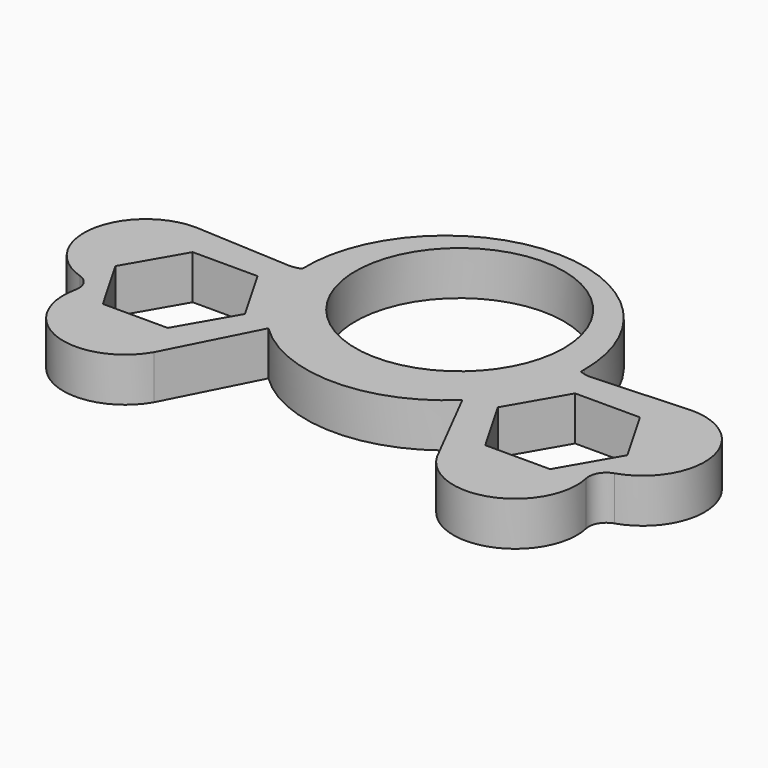
from build123d import *

# Parameters (mm, degrees)
F0_R     = 11.8128779822
F1_DEPTH = 5


with BuildPart() as f1:
    # F0 (on Top) → F1 (new body)
    with BuildSketch(Plane.XY):
        with BuildLine():
            ThreePointArc((-10.9877368692, -13.3584800376), (-14.4276328661, -8.4296575195), (-15.7757547816, -2.5722909453))
            ThreePointArc((-15.7757547816, -2.5722909453), (-16.4566838692, -2.7870228586), (-17.1690704864, -2.8347672253))
            Line((-17.1690704864, -2.8347672253), (-28.1587377075, -2.2588231712))
            ThreePointArc((-28.1587377075, -2.2588231712), (-35.0758085793, -8.184518487), (-30.2818924612, -15.9290715842))
            ThreePointArc((-30.2818924612, -15.9290715842), (-29.1564572976, -16.8348568451), (-28.9347418331, -18.2624049175))
            ThreePointArc((-28.9347418331, -18.2624049175), (-24.6247201691, -26.286334608), (-16.0343820545, -23.2588231712))
            Line((-16.0343820545, -23.2588231712), (-11.038330626, -13.4535201515))
            ThreePointArc((-11.038330626, -13.4535201515), (-11.0134601469, -13.4057731047), (-10.9877368692, -13.3584800376))
        make_face()
        Polygon((-29.0074426032, -12.5088231712), (-25.3354948912, -6.1488231712), (-17.9915994671, -6.1488231712), (-14.319651755, -12.5088231712), (-17.9915994671, -18.8688231712), (-25.3354948912, -18.8688231712), align=None, mode=Mode.SUBTRACT)
        with BuildLine():
            ThreePointArc((15.7758429715, -2.5697420135), (15.7828894553, -2.2975080655), (15.7852385163, -2.0251930691))
            ThreePointArc((15.7852385163, -2.0251930691), (13.4879848824, 6.1752958693), (7.264870736, 11.9889215374))
            ThreePointArc((7.264870736, 11.9889215374), (-8.4330311307, 11.3186347537), (-15.7757547816, -2.5722909453))
            ThreePointArc((-15.7757547816, -2.5722909453), (-14.4276328661, -8.4296575195), (-10.9877368692, -13.3584800376))
            ThreePointArc((-10.9877368692, -13.3584800376), (0.0010524985, -17.8104315503), (10.9892480908, -13.3570146974))
            ThreePointArc((10.9892480908, -13.3570146974), (14.4285771261, -8.4275299185), (15.7758429715, -2.5697420135))
        make_face()
        Circle(F0_R, mode=Mode.SUBTRACT)
        with BuildLine():
            ThreePointArc((17.1702555345, -2.8327146617), (16.4572773621, -2.784858795), (15.7758429715, -2.5697420135))
            ThreePointArc((15.7758429715, -2.5697420135), (14.4285771261, -8.4275299185), (10.9892480908, -13.3570146974))
            ThreePointArc((10.9892480908, -13.3570146974), (11.0148030033, -13.4040170233), (11.0395156741, -13.451467588))
            Line((11.0395156741, -13.451467588), (16.0355671026, -23.2567706076))
            ThreePointArc((16.0355671026, -23.2567706076), (24.6259052172, -26.2842820445), (28.9359268812, -18.260352354))
            ThreePointArc((28.9359268812, -18.260352354), (29.1576423457, -16.8328042815), (30.2830775093, -15.9270190207))
            ThreePointArc((30.2830775093, -15.9270190207), (35.0769936274, -8.1824659235), (28.1599227556, -2.2567706076))
            Line((28.1599227556, -2.2567706076), (17.1702555345, -2.8327146617))
        make_face()
        Polygon((25.3366799393, -18.8667706076), (17.9927845152, -18.8667706076), (14.3208368031, -12.5067706076), (17.9927845152, -6.1467706076), (25.3366799393, -6.1467706076), (29.0086276513, -12.5067706076), align=None, mode=Mode.SUBTRACT)
    extrude(amount=F1_DEPTH)


solid = f1.part
